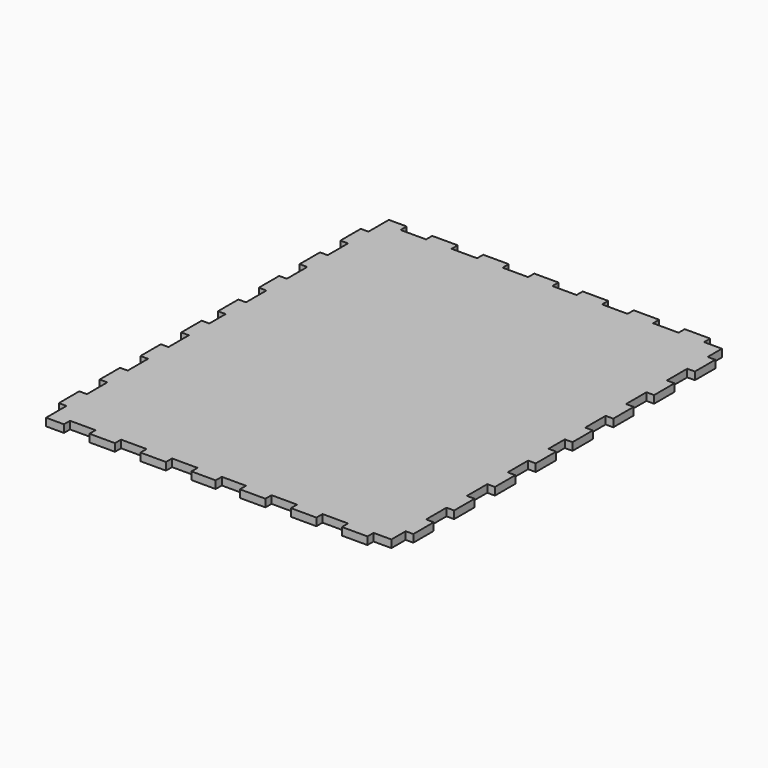
from build123d import *

# Parameters (mm, degrees)
F0_W     = 7
F0_H     = 3
F0_W_2   = 3
F0_H_2   = 10
F0_W_3   = 10
F0_W_4   = 9.5
F1_DEPTH = 1.5


with BuildPart() as f1:
    # F0 (on Top) → F1 (new body, symmetric)
    with BuildSketch(Plane.XY):
        with Locations((-63, 82.5)):
            Rectangle(F0_W, F0_H)
        Polygon((-59.5, 81), (-66.5, 81), (-66.5, 74), (-66.5, 64), (-66.5, 54), (-66.5, 44), (-66.5, 34), (-66.5, 24), (-66.5, 14), (-66.5, 4), (-66.5, 0), (0, 0), (0, 81), (-9.5, 81), (-19.5, 81), (-29.5, 81), (-39.5, 81), (-49.5, 81), align=None)
        with Locations((-68, 69)):
            Rectangle(F0_W_2, F0_H_2)
        with Locations((-44.5, 82.5)):
            Rectangle(F0_W_3, F0_H)
        with Locations((-68, 49)):
            Rectangle(F0_W_2, F0_H_2)
        with Locations((-24.5, 82.5)):
            Rectangle(F0_W_3, F0_H)
        with Locations((-68, 29)):
            Rectangle(F0_W_2, F0_H_2)
        with Locations((-4.75, 82.5)):
            Rectangle(F0_W_4, F0_H)
        with Locations((-68, 9)):
            Rectangle(F0_W_2, F0_H_2)
        Polygon((9.5, 81), (0, 81), (0, 0), (66.5, 0), (66.5, 4), (66.5, 14), (66.5, 24), (66.5, 34), (66.5, 44), (66.5, 54), (66.5, 64), (66.5, 74), (66.5, 81), (59.5, 81), (49.5, 81), (39.5, 81), (29.5, 81), (19.5, 81), align=None)
        with Locations((14.5, 82.5)):
            Rectangle(F0_W_3, F0_H)
        Polygon((0, -81), (0, 0), (-66.5, 0), (-66.5, -4), (-66.5, -14), (-66.5, -24), (-66.5, -34), (-66.5, -44), (-66.5, -54), (-66.5, -64), (-66.5, -74), (-66.5, -81), (-59.5, -81), (-49.5, -81), (-39.5, -81), (-29.5, -81), (-19.5, -81), (-9.5, -81), align=None)
        Polygon((66.5, 0), (0, 0), (0, -81), (9.5, -81), (19.5, -81), (29.5, -81), (39.5, -81), (49.5, -81), (59.5, -81), (66.5, -81), (66.5, -74), (66.5, -64), (66.5, -54), (66.5, -44), (66.5, -34), (66.5, -24), (66.5, -14), (66.5, -4), align=None)
        with Locations((-4.75, -82.5)):
            Rectangle(F0_W_4, F0_H)
        with Locations((34.5, 82.5)):
            Rectangle(F0_W_3, F0_H)
        with Locations((-68, -9)):
            Rectangle(F0_W_2, F0_H_2)
        with Locations((68, 9)):
            Rectangle(F0_W_2, F0_H_2)
        with Locations((68, -9)):
            Rectangle(F0_W_2, F0_H_2)
        with Locations((14.5, -82.5)):
            Rectangle(F0_W_3, F0_H)
        with Locations((-24.5, -82.5)):
            Rectangle(F0_W_3, F0_H)
        with Locations((54.5, 82.5)):
            Rectangle(F0_W_3, F0_H)
        with Locations((-68, -29)):
            Rectangle(F0_W_2, F0_H_2)
        with Locations((68, 29)):
            Rectangle(F0_W_2, F0_H_2)
        with Locations((68, -29)):
            Rectangle(F0_W_2, F0_H_2)
        with Locations((34.5, -82.5)):
            Rectangle(F0_W_3, F0_H)
        with Locations((-44.5, -82.5)):
            Rectangle(F0_W_3, F0_H)
        with Locations((-68, -49)):
            Rectangle(F0_W_2, F0_H_2)
        with Locations((68, 49)):
            Rectangle(F0_W_2, F0_H_2)
        with Locations((68, -49)):
            Rectangle(F0_W_2, F0_H_2)
        with Locations((54.5, -82.5)):
            Rectangle(F0_W_3, F0_H)
        with Locations((-63, -82.5)):
            Rectangle(F0_W, F0_H)
        with Locations((68, 69)):
            Rectangle(F0_W_2, F0_H_2)
        with Locations((-68, -69)):
            Rectangle(F0_W_2, F0_H_2)
        with Locations((68, -69)):
            Rectangle(F0_W_2, F0_H_2)
    extrude(amount=F1_DEPTH, both=True)


solid = f1.part
